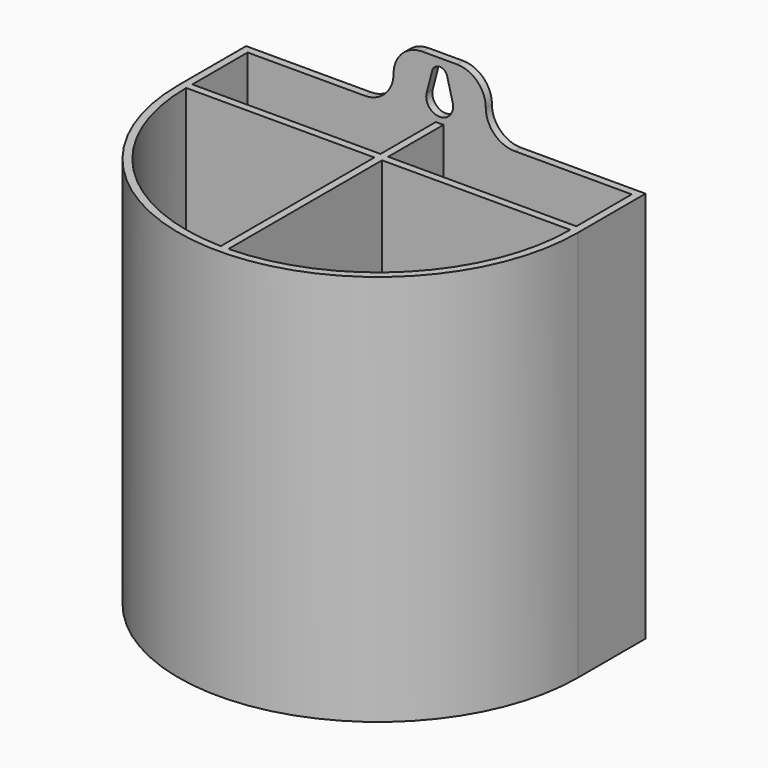
from build123d import *

# Parameters (mm, degrees)
F1_DEPTH = 2
F2_W     = 49
F2_H     = 18
F3_DEPTH = 100
F4_W     = 24
F4_H     = 2
F5_DEPTH = 15
F7_DEPTH = 2
F8_R     = 7.49999


# Not quite as in the source:
# - a fillet or chamfer is up to 0.001 mm smaller than in the source, because OpenCascade refuses the exact size


with BuildPart() as f1:
    # F0 (on Top) → F1 (new body)
    with BuildSketch(Plane.XY):
        with BuildLine():
            Line((104, 0), (0, 0))
            Line((0, 0), (0, -22))
            ThreePointArc((0, -22), (52, -74), (104, -22))
            Line((104, -22), (104, 0))
        make_face()
    extrude(amount=F1_DEPTH)

    # F2 (on face) → F3 (join)
    with BuildSketch(Plane.XY.offset(2)):
        with BuildLine():
            Line((104, 0), (0, 0))
            Line((0, 0), (0, -22))
            ThreePointArc((0, -22), (52, -74), (104, -22))
            Line((104, -22), (104, 0))
        make_face()
        with BuildLine():
            ThreePointArc((51, -71.9899989998), (16.2928578573, -57), (2, -22))
            Line((2, -22), (51, -22))
            Line((51, -22), (51, -71.9899989998))
        make_face(mode=Mode.SUBTRACT)
        with BuildLine():
            ThreePointArc((102, -22), (87.7071421427, -57), (53, -71.9899989998))
            Line((53, -71.9899989998), (53, -22))
            Line((53, -22), (102, -22))
        make_face(mode=Mode.SUBTRACT)
        with Locations((26.5, -11)):
            Rectangle(F2_W, F2_H, mode=Mode.SUBTRACT)
        with Locations((77.5, -11)):
            Rectangle(F2_W, F2_H, mode=Mode.SUBTRACT)
    extrude(amount=F3_DEPTH)

    # F4 (on face) → F5 (join)
    with BuildSketch(Plane.XY.offset(102)):
        with Locations((52, -1)):
            Rectangle(F4_W, F4_H)
    extrude(amount=F5_DEPTH)

    # F6 (on face) → F7 (cut, through all)
    with BuildSketch(Plane.XZ.offset(2)):
        with BuildLine():
            Line((55.3888604279, 107.875), (53.9364916731, 113.5))
            ThreePointArc((53.9364916731, 113.5), (52, 115), (50.0635083269, 113.5))
            Line((50.0635083269, 113.5), (48.6111395721, 107.875))
            ThreePointArc((48.6111395721, 107.875), (52, 103.5), (55.3888604279, 107.875))
        make_face()
    extrude(amount=-F7_DEPTH, mode=Mode.SUBTRACT)

    # F8 (radius 7.5 in the source; OpenCascade refuses exactly that, so slightly less here)
    f8_edges = [f1.edges().sort_by_distance(p)[0] for p in [
        (64, -1, 102),
        (64, -1, 117),
        (40, -1, 102),
        (40, -1, 117),
    ]]
    fillet(f8_edges, radius=F8_R)


solid = f1.part
